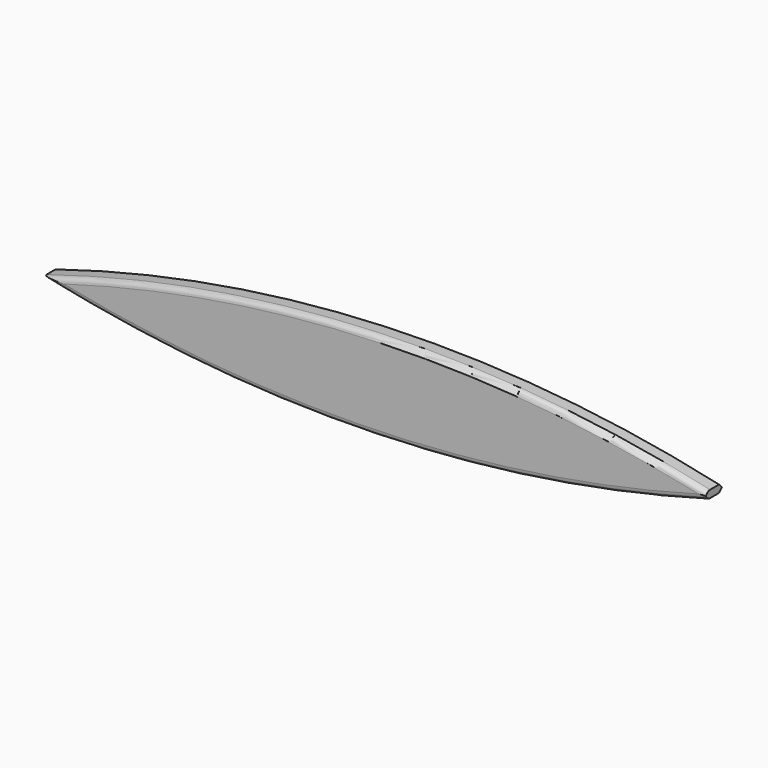
from build123d import *

# Parameters (mm, degrees)
F1_DEPTH    = 127
F2_T2_ANGLE = 31.186938852
F2_T4_ANGLE = 29.2868339597
F3_C1_SIZE  = 88.9
F3_C2_SIZE  = 88.9


# Not quite as in the source:
# - a fillet or chamfer that OpenCascade refuses, or shapes differently, is made with other operations: its cross-section is extruded or revolved along the edge and cut away or added


with BuildPart() as f1:
    # F0 (on Front) → F1 (new body)
    with BuildSketch(Plane.XZ):
        with BuildLine():
            Line((1083.5856187426, 43.4364019366), (1083.5856187426, 60.5836437908))
            ThreePointArc((1083.5856187426, 60.5836437908), (317.5983414893, 130.5929948501), (-440.4143812574, 0))
            ThreePointArc((-440.4143812574, 0), (324.2681839508, -72.4016891466), (1083.5856187426, 43.4364019366))
        make_face()
    extrude(amount=F1_DEPTH)

    # F2: fillet of radius 12.2642048969 on 3 edges, made by hand

    # F2_s1 → F2_t2 (revolve, cut)
    with BuildSketch(Plane(origin=(1042.3525858454, 0, -246.7280237768), x_dir=(0, 1, 0), z_dir=(0.973110628, 0, -0.230338242))):
        with BuildLine():
            ThreePointArc((-114.7357951031, 308.7053036416), (-123.4078975516, 305.1132011932), (-127, 296.4410987447))
            Line((-127, 296.4410987447), (-127, 308.7053036416))
            Line((-127, 308.7053036416), (-114.7357951031, 308.7053036416))
        make_face()
    revolve(axis=Axis((434.657275986, -127, -2814.0601328001), (0, -1, 0)), revolution_arc=F2_T2_ANGLE, mode=Mode.SUBTRACT)

    # F2_s3 → F2_t4 (revolve, cut)
    with BuildSketch(Plane(origin=(-447.9656433365, 0, 103.5102824727), x_dir=(0, 1, 0), z_dir=(-0.9743274922, 0, 0.2251353769))):
        with BuildLine():
            ThreePointArc((-114.7357951031, 99.3028983442), (-123.4078975516, 95.7107958958), (-127, 87.0386934473))
            Line((-127, 87.0386934473), (-127, 99.3028983442))
            Line((-127, 99.3028983442), (-114.7357951031, 99.3028983442))
        make_face()
    revolve(axis=Axis((235.0110043049, -127, 3059.2559923266), (0, -1, 0)), revolution_arc=F2_T4_ANGLE, mode=Mode.SUBTRACT)

    # F3: chamfer of 88.9 on 2 edges, made by hand

    # F3_c1
    f3_c1_edges = [f1.edges().sort_by_distance(p)[0] for p in [
        (317.5983414893, 0, 130.5929948501),
    ]]
    chamfer(f3_c1_edges, length=F3_C1_SIZE)

    # F3_c2
    f3_c2_edges = [f1.edges().sort_by_distance(p)[0] for p in [
        (341.4443406907, 0, -71.8649927128),
    ]]
    chamfer(f3_c2_edges, length=F3_C2_SIZE)


solid = f1.part
